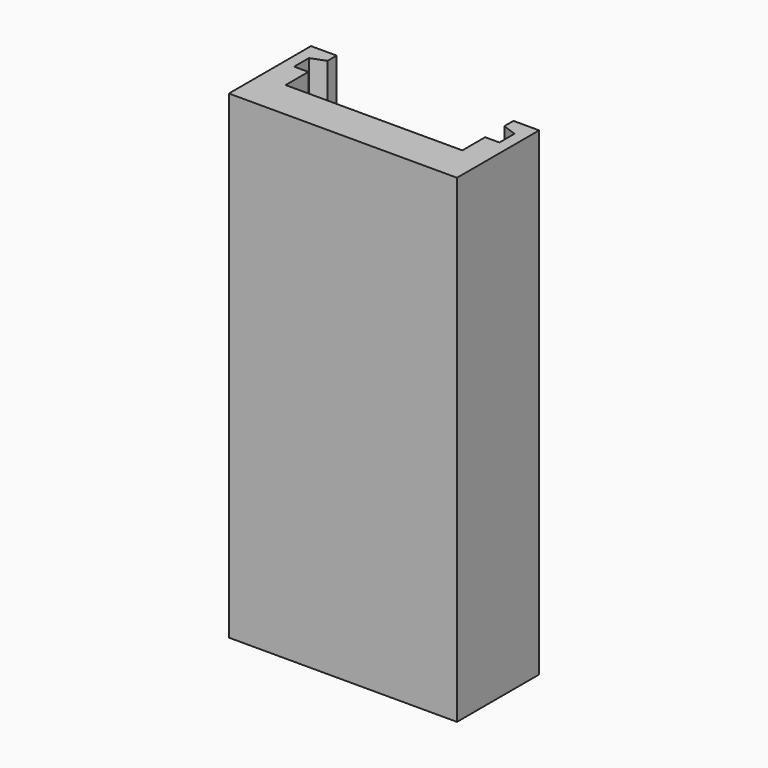
from build123d import *

# Parameters (mm, degrees)
F0_W        = 20
F0_H        = 42
F1_DEPTH    = 9
F2_W        = 15.5
F2_H        = 1.5
F2_H_2      = 1.6
F2_W_2      = 1.25
F2_H_3      = 2.5
F3_DEPTH    = 42.001
F4_T4_DEPTH = 48.7433158126
F5_T4_DEPTH = 49.2642981969


# Not quite as in the source:
# - a fillet or chamfer that OpenCascade refuses, or shapes differently, is made with other operations: its cross-section is extruded or revolved along the edge and cut away or added


with BuildPart() as f1:
    # F0 (on Front) → F1 (new body)
    with BuildSketch(Plane.XZ):
        Rectangle(F0_W, F0_H)
    extrude(amount=F1_DEPTH)

    # F2 (on face) → F3 (cut, through all)
    with BuildSketch(Plane.XY.offset(21)):
        with Locations((0, -0.75)):
            Rectangle(F2_W, F2_H)
        with Locations((0, -2.3)):
            Rectangle(F2_W, F2_H_2)
        with Locations((-8.375, -2.3)):
            Rectangle(F2_W_2, F2_H_2)
        with Locations((8.375, -2.3)):
            Rectangle(F2_W_2, F2_H_2)
        with Locations((0, -4.35)):
            Rectangle(F2_W, F2_H_3)
    extrude(amount=-F3_DEPTH, mode=Mode.SUBTRACT)

    # F4: chamfer of 1.3 x 0.5 on 1 edges, made by hand


with BuildPart() as f4_tool2:
    # F4_s3 → F4_t4 (new body)
    with BuildSketch(Plane.XY.offset(24.3716579063)):
        Polygon((-7.75, -1), (-9.05, -1.5), (-7.75, -1.5), align=None)
    extrude(amount=-F4_T4_DEPTH)

    split(bisect_by=Plane.YZ.offset(-9), keep=Keep.TOP)


with BuildPart() as f1_1:
    add(f1.part)

    # F4_t1: cut F4_tool2
    add(f4_tool2.part, mode=Mode.SUBTRACT)

    # F5: chamfer of 1.4 x 0.5 on 1 edges, made by hand


with BuildPart() as f5_tool2:
    # F5_s3 → F5_t4 (new body)
    with BuildSketch(Plane.XY.offset(24.6321490984)):
        Polygon((9.15, -1.5), (7.75, -1), (7.75, -1.5), align=None)
    extrude(amount=-F5_T4_DEPTH)

    split(bisect_by=Plane.YZ.offset(9), keep=Keep.BOTTOM)


with BuildPart() as f1_2:
    add(f1_1.part)

    # F5_t1: cut F5_tool2
    add(f5_tool2.part, mode=Mode.SUBTRACT)


solid = f1_2.part
